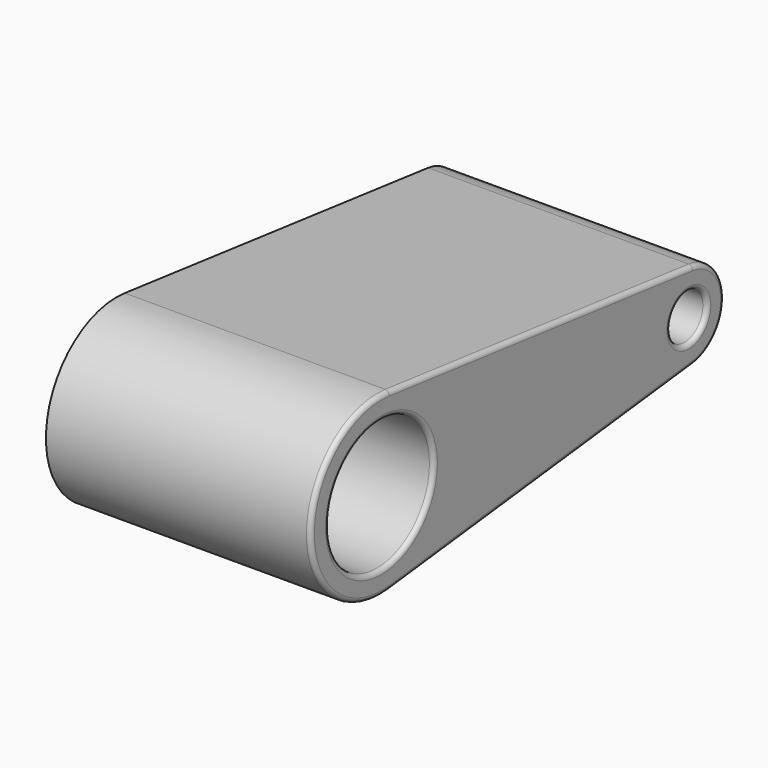
from build123d import *

# Parameters (mm, degrees)
F1_DEPTH    = 76.2
F2_R        = 18.8420717169
F2_R_2      = 6.614317189
F3_DEPTH    = 50.8
F4_R        = 1.27
F5_T        = -2.54
F6_R        = 1.27
F7_R        = 1.27
F8_T1_DEPTH = 109.83255313
F8_T3_DEPTH = 109.83255313
F8_T6_ANGLE = 193.1917018044
F8_T8_ANGLE = 166.8082981956


# Not quite as in the source:
# - a fillet or chamfer that OpenCascade refuses, or shapes differently, is made with other operations: its cross-section is extruded or revolved along the edge and cut away or added


with BuildPart() as f1:
    # F0 (on Right) → F1 (new body)
    with BuildSketch(Plane.YZ):
        with BuildLine():
            ThreePointArc((2.9175764531, -25.2318795899), (18.9639980214, -16.8975376622), (25.4, 0))
            ThreePointArc((25.4, 0), (18.9639980214, 16.8975376622), (2.9175764531, 25.2318795899))
            ThreePointArc((2.9175764531, 25.2318795899), (-25.4, 0), (2.9175764531, -25.2318795899))
        make_face()
        with BuildLine():
            ThreePointArc((2.9175764531, 25.2318795899), (18.9639980214, 16.8975376622), (25.4, 0))
            ThreePointArc((25.4, 0), (18.9639980214, -16.8975376622), (2.9175764531, -25.2318795899))
            Line((2.9175764531, -25.2318795899), (112.0231573834, -12.615939795))
            ThreePointArc((112.0231573834, -12.615939795), (97.8643691568, 0), (112.0231573834, 12.615939795))
            Line((112.0231573834, 12.615939795), (2.9175764531, 25.2318795899))
        make_face()
        with BuildLine():
            ThreePointArc((123.2643691568, 0), (120.0463681675, 8.4487688311), (112.0231573834, 12.615939795))
            ThreePointArc((112.0231573834, 12.615939795), (97.8643691568, 0), (112.0231573834, -12.615939795))
            ThreePointArc((112.0231573834, -12.615939795), (120.0463681675, -8.4487688311), (123.2643691568, 0))
        make_face()
    extrude(amount=F1_DEPTH)

    # F2 (on face) → F3 (cut)
    with BuildSketch(Plane.YZ.offset(76.2)):
        Circle(F2_R)
        with Locations((110.5643691568, 0)):
            Circle(F2_R_2)
    extrude(amount=-F3_DEPTH, mode=Mode.SUBTRACT)

    # F4
    f4_edges = [f1.edges().sort_by_distance(p)[0] for p in [
        (76.2, -25.4, 0),
        (76.2, -18.842072, 0),
        (76.2, 103.950052, 0),
    ]]
    fillet(f4_edges, radius=F4_R)

    # F5
    f5_openings = [f1.faces().sort_by_distance(p)[0] for p in [
        (0, 41.190911, 0),
    ]]
    offset(amount=F5_T, openings=f5_openings, kind=Kind.INTERSECTION)

    # F6
    f6_edges = [f1.edges().sort_by_distance(p)[0] for p in [
        (0, 57.178609, 16.400722),
    ]]
    fillet(f6_edges, radius=F6_R)

    # F7
    f7_edges = [f1.edges().sort_by_distance(p)[0] for p in [
        (22.86, 101.410052, 0),
        (48.26, 119.718686, 0),
    ]]
    fillet(f7_edges, radius=F7_R)

    # F8: fillet of radius 1.27 on 8 edges, made by hand

    # F8_s2 → F8_t1 (join)
    with BuildSketch(Plane(origin=(0, 109.1055809303, -12.615939795), x_dir=(1, 0, 0), z_dir=(0, -0.9933810862, 0.1148652147))):
        with BuildLine():
            ThreePointArc((73.6604, 21.5890343146), (73.2880256121, 22.4880256121), (72.3890343146, 22.8604))
            Line((72.3890343146, 22.8604), (72.3890343146, 22.9875365685))
            ThreePointArc((72.3890343146, 22.9875365685), (73.0245171573, 22.9871365685), (73.66, 22.9871365685))
            Line((73.66, 22.9871365685), (73.7871365685, 22.86))
            ThreePointArc((73.7871365685, 22.86), (73.7871365685, 22.2245171573), (73.7875365685, 21.5890343146))
            Line((73.7875365685, 21.5890343146), (73.6604, 21.5890343146))
        make_face()
    extrude(amount=F8_T1_DEPTH)

    # F8_s4 → F8_t3 (join)
    with BuildSketch(Plane(origin=(0, 0, 0), x_dir=(1, 0, 0), z_dir=(0, 0.9933810862, 0.1148652147))):
        with BuildLine():
            ThreePointArc((73.6604, 21.5890343146), (73.2880256121, 22.4880256121), (72.3890343146, 22.8604))
            Line((72.3890343146, 22.8604), (72.3890343146, 22.9875365685))
            ThreePointArc((72.3890343146, 22.9875365685), (73.0245171573, 22.9871365685), (73.66, 22.9871365685))
            Line((73.66, 22.9871365685), (73.7871365685, 22.86))
            ThreePointArc((73.7871365685, 22.86), (73.7871365685, 22.2245171573), (73.7875365685, 21.5890343146))
            Line((73.7875365685, 21.5890343146), (73.6604, 21.5890343146))
        make_face()
    extrude(amount=F8_T3_DEPTH)

    # F8_s5 → F8_t6 (revolve)
    with BuildSketch(Plane(origin=(0, 0, 0), x_dir=(1, 0, 0), z_dir=(0, 0.9933810862, 0.1148652147))):
        with BuildLine():
            ThreePointArc((73.6604, 21.5890343146), (73.2880256121, 22.4880256121), (72.3890343146, 22.8604))
            Line((72.3890343146, 22.8604), (72.3890343146, 22.9875365685))
            ThreePointArc((72.3890343146, 22.9875365685), (73.0245171573, 22.9871365685), (73.66, 22.9871365685))
            Line((73.66, 22.9871365685), (73.7871365685, 22.86))
            ThreePointArc((73.7871365685, 22.86), (73.7871365685, 22.2245171573), (73.7875365685, 21.5890343146))
            Line((73.7875365685, 21.5890343146), (73.6604, 21.5890343146))
        make_face()
    revolve(axis=Axis((73.66, 0, 0), (-1, 0, 0)), revolution_arc=F8_T6_ANGLE)

    # F8_s7 → F8_t8 (revolve)
    with BuildSketch(Plane(origin=(0, 109.1055809303, -12.615939795), x_dir=(1, 0, 0), z_dir=(0, -0.9933810862, 0.1148652147))):
        with BuildLine():
            ThreePointArc((73.6604, 21.5890343146), (73.2880256121, 22.4880256121), (72.3890343146, 22.8604))
            Line((72.3890343146, 22.8604), (72.3890343146, 22.9875365685))
            ThreePointArc((72.3890343146, 22.9875365685), (73.0245171573, 22.9871365685), (73.66, 22.9871365685))
            Line((73.66, 22.9871365685), (73.7871365685, 22.86))
            ThreePointArc((73.7871365685, 22.86), (73.7871365685, 22.2245171573), (73.7875365685, 21.5890343146))
            Line((73.7875365685, 21.5890343146), (73.6604, 21.5890343146))
        make_face()
    revolve(axis=Axis((73.66, 110.5643691568, 0), (-1, 0, 0)), revolution_arc=F8_T8_ANGLE)

    # F8_s9 → F8_t10 (revolve)
    with BuildSketch(Plane.XY):
        with BuildLine():
            ThreePointArc((72.3890343146, 119.7182863458), (73.2880256121, 120.0906607337), (73.6604, 120.9896520312))
            Line((73.6604, 120.9896520312), (73.7875365685, 120.9896520312))
            ThreePointArc((73.7875365685, 120.9896520312), (73.7871365685, 120.3541691885), (73.7871365685, 119.7186863458))
            Line((73.7871365685, 119.7186863458), (73.66, 119.5915497773))
            ThreePointArc((73.66, 119.5915497773), (73.0245171573, 119.5915497773), (72.3890343146, 119.5911497773))
            Line((72.3890343146, 119.5911497773), (72.3890343146, 119.7182863458))
        make_face()
    revolve(axis=Axis((73.66, 110.5643691568, 0), (1, 0, 0)))

    # F8_s11 → F8_t12 (revolve)
    with BuildSketch(Plane.XY):
        with BuildLine():
            ThreePointArc((73.6604, 22.6530374023), (73.2880256121, 21.7540461048), (72.3890343146, 21.3816717169))
            Line((72.3890343146, 21.3816717169), (72.3890343146, 21.2545351484))
            ThreePointArc((72.3890343146, 21.2545351484), (73.0245171573, 21.2549351484), (73.66, 21.2549351484))
            Line((73.66, 21.2549351484), (73.7871365685, 21.3820717169))
            ThreePointArc((73.7871365685, 21.3820717169), (73.7871365685, 22.0175545596), (73.7875365685, 22.6530374023))
            Line((73.7875365685, 22.6530374023), (73.6604, 22.6530374023))
        make_face()
    revolve(axis=Axis((73.66, 0, 0), (1, 0, 0)))

    # F8_s13 → F8_t14 (revolve, cut)
    with BuildSketch(Plane.XY):
        with BuildLine():
            ThreePointArc((24.1309656854, 21.3824717169), (23.2319743879, 21.010097329), (22.8596, 20.1111060315))
            Line((22.8596, 20.1111060315), (22.7324634315, 20.1111060315))
            ThreePointArc((22.7324634315, 20.1111060315), (22.7328634315, 20.7465888742), (22.7328634315, 21.3820717169))
            Line((22.7328634315, 21.3820717169), (22.86, 21.5092082855))
            ThreePointArc((22.86, 21.5092082855), (23.4954828427, 21.5092082855), (24.1309656854, 21.5096082855))
            Line((24.1309656854, 21.5096082855), (24.1309656854, 21.3824717169))
        make_face()
    revolve(axis=Axis((22.86, 0, 0), (1, 0, 0)), mode=Mode.SUBTRACT)


solid = f1.part
